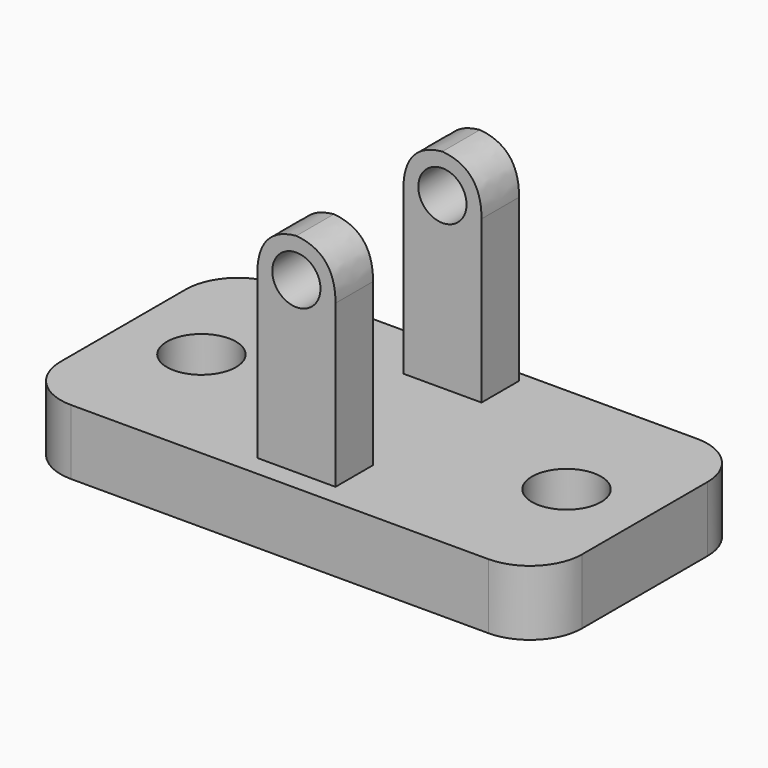
from build123d import *

# Parameters (mm, degrees)
F0_W        = 50.8
F0_H        = 25.4
F0_R        = 3.3655
F1_DEPTH    = 6.35
F2_R        = 5.08
F3_W        = 7.62
F3_H        = 4.572
F4_DEPTH    = 20.32
F5_R        = 2.3495
F6_DEPTH    = 25.4
F7_T1_DEPTH = 27.432
F7_T3_DEPTH = 27.432


# Not quite as in the source:
# - a fillet or chamfer that OpenCascade refuses, or shapes differently, is made with other operations: its cross-section is extruded or revolved along the edge and cut away or added


with BuildPart() as f1:
    # F0 (on Top) → F1 (new body)
    with BuildSketch(Plane.XY):
        with Locations((14.6050021708, 1.6630402533)):
            Rectangle(F0_W, F0_H)
        with Locations((-3.1749978292, 1.6630402533)):
            Circle(F0_R, mode=Mode.SUBTRACT)
        with Locations((32.3850021708, 1.6630402533)):
            Circle(F0_R, mode=Mode.SUBTRACT)
    extrude(amount=F1_DEPTH)

    # F2
    f2_edges = [f1.edges().sort_by_distance(p)[0] for p in [
        (40.005002, -11.03696, 3.175),
        (40.005002, 14.36304, 3.175),
        (-10.794998, -11.03696, 3.175),
        (-10.794998, 14.36304, 3.175),
    ]]
    fillet(f2_edges, radius=F2_R)

    # F3 (on face) → F4 (join)
    with BuildSketch(Plane.XY.offset(6.35)):
        with Locations((14.6050021708, 11.0610402533)):
            Rectangle(F3_W, F3_H)
        with Locations((14.6050021708, -6.7189597467)):
            Rectangle(F3_W, F3_H)
    extrude(amount=F4_DEPTH)

    # F5 (on face) → F6 (cut)
    with BuildSketch(Plane(origin=(0, 13.3470402533, 0), x_dir=(-1, 0, 0), z_dir=(0, 1, 0))):
        with Locations((-14.6050021708, 22.86)):
            Circle(F5_R)
    extrude(amount=-F6_DEPTH, mode=Mode.SUBTRACT)

    # F7: fillet of radius 4.572 on 4 edges, made by hand

    # F7_s2 → F7_t1 (cut)
    with BuildSketch(Plane.XZ.offset(-6.9970402533)):
        with BuildLine():
            add(Edge.make_bspline(
                [(18.4150021708, 22.098), (18.4150021708, 26.67), (13.8430021708, 26.67)],
                knots=[0, 0, 0, 1, 1, 1], degree=2, weights=[1, 1, 1]))
            Line((13.8430021708, 26.67), (18.4150021708, 26.67))
            Line((18.4150021708, 26.67), (18.4150021708, 22.098))
        make_face()
        with BuildLine():
            add(Edge.make_bspline(
                [(10.7950021708, 22.098), (10.7950021708, 26.67), (15.3670021708, 26.67)],
                knots=[0, 0, 0, 1, 1, 1], degree=2, weights=[1, 1, 1]))
            Line((15.3670021708, 26.67), (10.7950021708, 26.67))
            Line((10.7950021708, 26.67), (10.7950021708, 22.098))
        make_face()
    extrude(amount=F7_T1_DEPTH, mode=Mode.SUBTRACT)

    # F7_s4 → F7_t3 (cut)
    with BuildSketch(Plane.XZ.offset(-24.7770402533)):
        with BuildLine():
            add(Edge.make_bspline(
                [(18.4150021708, 22.098), (18.4150021708, 26.67), (13.8430021708, 26.67)],
                knots=[0, 0, 0, 1, 1, 1], degree=2, weights=[1, 1, 1]))
            Line((13.8430021708, 26.67), (18.4150021708, 26.67))
            Line((18.4150021708, 26.67), (18.4150021708, 22.098))
        make_face()
        with BuildLine():
            add(Edge.make_bspline(
                [(10.7950021708, 22.098), (10.7950021708, 26.67), (15.3670021708, 26.67)],
                knots=[0, 0, 0, 1, 1, 1], degree=2, weights=[1, 1, 1]))
            Line((15.3670021708, 26.67), (10.7950021708, 26.67))
            Line((10.7950021708, 26.67), (10.7950021708, 22.098))
        make_face()
    extrude(amount=F7_T3_DEPTH, mode=Mode.SUBTRACT)


solid = f1.part
